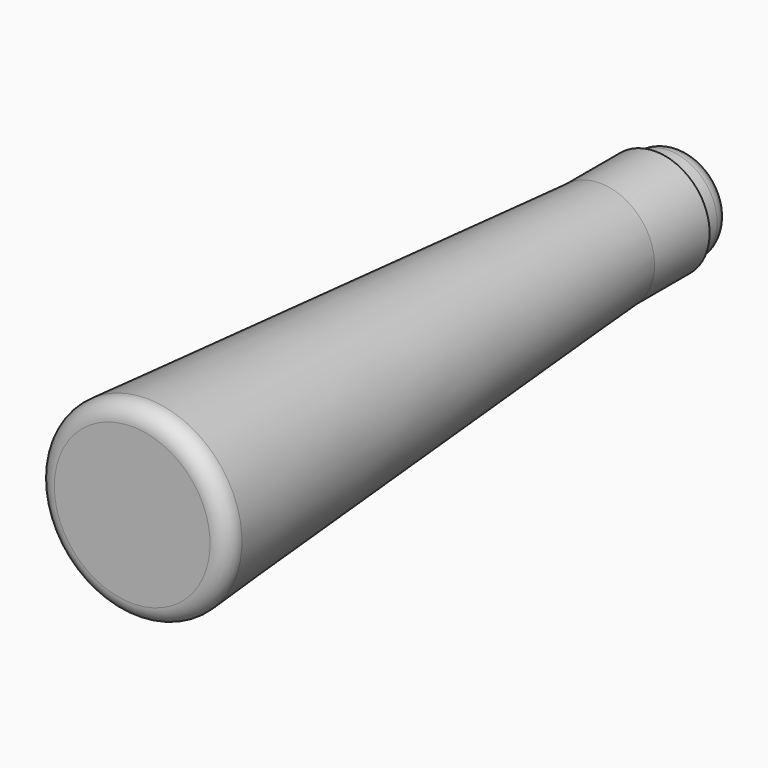
from build123d import *

# Parameters (mm, degrees)
F2_R     = 5
F3_DEPTH = 20
F4_R     = 14
F5_DEPTH = 10
F6_R     = 5


with BuildPart() as f1:
    # F0 (on Top) → F1 (revolve)
    with BuildSketch(Plane.XY):
        Polygon((12.2, 170), (0, 0), (28, 0), (28, 170), align=None)
    revolve(axis=Axis((28, 85, 0), (0, 1, 0)))

    # F2
    f2_edges = [f1.edges().sort_by_distance(p)[0] for p in [
        (56, 0, 0),
    ]]
    fillet(f2_edges, radius=F2_R)


with BuildPart() as f3:
    # F3 (new): a face of the model
    f3_faces = [f1.part.faces().sort_by_distance(p)[0] for p in [
        (28, 170, 0),
    ]]
    extrude(f3_faces, amount=F3_DEPTH)


with BuildPart() as f5:
    # F4 (on face) → F5 (new body)
    with BuildSketch(Plane(origin=(0, 190, 0), x_dir=(-1, 0, 0), z_dir=(0, 1, 0))):
        with Locations((-28, 0)):
            Circle(F4_R)
    extrude(amount=F5_DEPTH)

    # F6
    f6_edges = [f5.edges().sort_by_distance(p)[0] for p in [
        (42, 200, 0),
    ]]
    fillet(f6_edges, radius=F6_R)


solid = Compound([f1.part, f3.part, f5.part])
